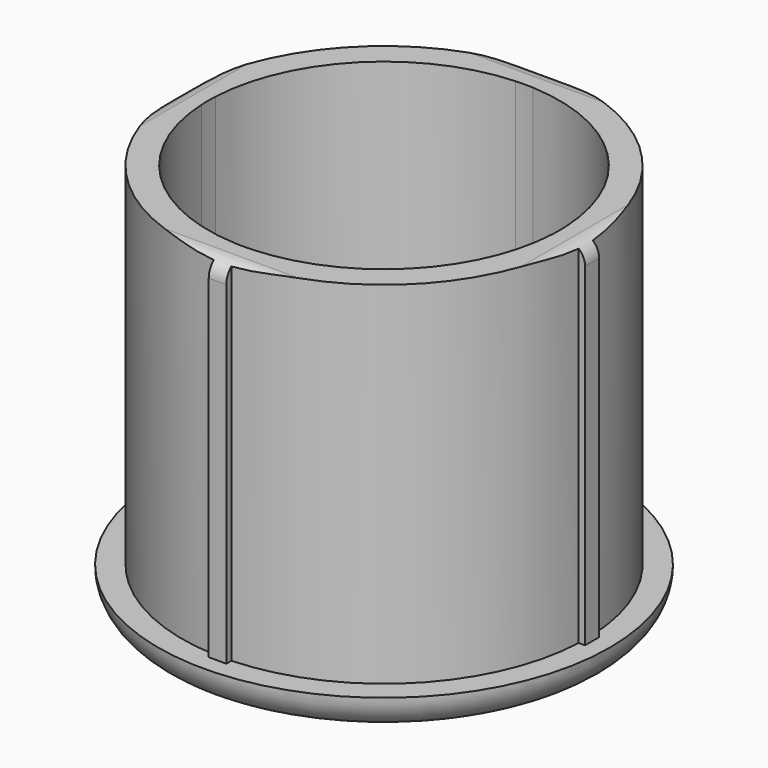
from build123d import *

# Parameters (mm, degrees)
F0_R     = 12.85
F1_DEPTH = 2
F3_DEPTH = 20
F4_R     = 1
F5_R     = 1.99999


# Not quite as in the source:
# - a fillet or chamfer is up to 0.001 mm smaller than in the source, because OpenCascade refuses the exact size


with BuildPart() as f1:
    # F0 (on Top) → F1 (new body)
    with BuildSketch(Plane.XY):
        Circle(F0_R)
    extrude(amount=F1_DEPTH)

    # F2 (on face) → F3 (join)
    with BuildSketch(Plane.XY.offset(2)):
        with BuildLine():
            ThreePointArc((11.4891252931, -0.5), (11.4972810018, -0.2500591226), (11.5, 0))
            ThreePointArc((11.5, 0), (11.4972810018, 0.2500591226), (11.4891252931, 0.5))
            Line((11.4891252931, 0.5), (9.9874921777, 0.5))
            ThreePointArc((9.9874921777, 0.5), (9.9968725554, 0.2500782106), (10, 0))
            ThreePointArc((10, 0), (9.9968725554, -0.2500782106), (9.9874921777, -0.5))
            Line((9.9874921777, -0.5), (11.4891252931, -0.5))
        make_face()
        with BuildLine():
            ThreePointArc((11.4891252931, 0.5), (11.4972810018, 0.2500591226), (11.5, 0))
            ThreePointArc((11.5, 0), (11.4972810018, -0.2500591226), (11.4891252931, -0.5))
            Line((11.4891252931, -0.5), (11.85, -0.5))
            Line((11.85, -0.5), (11.85, 0.5))
            Line((11.85, 0.5), (11.4891252931, 0.5))
        make_face()
        with BuildLine():
            Line((9.9874921777, 0.5), (11.4891252931, 0.5))
            ThreePointArc((11.4891252931, 0.5), (8.1317279836, 8.1317279836), (0.5, 11.4891252931))
            Line((0.5, 11.4891252931), (0.5, 9.9874921777))
            ThreePointArc((0.5, 9.9874921777), (7.0710678119, 7.0710678119), (9.9874921777, 0.5))
        make_face()
        with BuildLine():
            ThreePointArc((0.5, -11.4891252931), (8.1317279836, -8.1317279836), (11.4891252931, -0.5))
            Line((11.4891252931, -0.5), (9.9874921777, -0.5))
            ThreePointArc((9.9874921777, -0.5), (7.0710678119, -7.0710678119), (0.5, -9.9874921777))
            Line((0.5, -9.9874921777), (0.5, -11.4891252931))
        make_face()
        with BuildLine():
            Line((0.5, 9.9874921777), (0.5, 11.4891252931))
            ThreePointArc((0.5, 11.4891252931), (0, 11.5), (-0.5, 11.4891252931))
            Line((-0.5, 11.4891252931), (-0.5, 9.9874921777))
            ThreePointArc((-0.5, 9.9874921777), (0, 10), (0.5, 9.9874921777))
        make_face()
        with BuildLine():
            ThreePointArc((-0.5, 11.4891252931), (0, 11.5), (0.5, 11.4891252931))
            Line((0.5, 11.4891252931), (0.5, 11.85))
            Line((0.5, 11.85), (-0.5, 11.85))
            Line((-0.5, 11.85), (-0.5, 11.4891252931))
        make_face()
        with BuildLine():
            Line((0.5, -11.85), (0.5, -11.4891252931))
            ThreePointArc((0.5, -11.4891252931), (0, -11.5), (-0.5, -11.4891252931))
            Line((-0.5, -11.4891252931), (-0.5, -11.85))
            Line((-0.5, -11.85), (0.5, -11.85))
        make_face()
        with BuildLine():
            ThreePointArc((-0.5, -11.4891252931), (0, -11.5), (0.5, -11.4891252931))
            Line((0.5, -11.4891252931), (0.5, -9.9874921777))
            ThreePointArc((0.5, -9.9874921777), (0, -10), (-0.5, -9.9874921777))
            Line((-0.5, -9.9874921777), (-0.5, -11.4891252931))
        make_face()
        with BuildLine():
            Line((-0.5, 9.9874921777), (-0.5, 11.4891252931))
            ThreePointArc((-0.5, 11.4891252931), (-8.1317279836, 8.1317279836), (-11.4891252931, 0.5))
            Line((-11.4891252931, 0.5), (-9.9874921777, 0.5))
            ThreePointArc((-9.9874921777, 0.5), (-7.0710678119, 7.0710678119), (-0.5, 9.9874921777))
        make_face()
        with BuildLine():
            ThreePointArc((-11.4891252931, -0.5), (-8.1317279836, -8.1317279836), (-0.5, -11.4891252931))
            Line((-0.5, -11.4891252931), (-0.5, -9.9874921777))
            ThreePointArc((-0.5, -9.9874921777), (-7.0710678119, -7.0710678119), (-9.9874921777, -0.5))
            Line((-9.9874921777, -0.5), (-11.4891252931, -0.5))
        make_face()
        with BuildLine():
            Line((-9.9874921777, 0.5), (-11.4891252931, 0.5))
            ThreePointArc((-11.4891252931, 0.5), (-11.5, 0), (-11.4891252931, -0.5))
            Line((-11.4891252931, -0.5), (-9.9874921777, -0.5))
            ThreePointArc((-9.9874921777, -0.5), (-10, 0), (-9.9874921777, 0.5))
        make_face()
        with BuildLine():
            ThreePointArc((-11.4891252931, -0.5), (-11.5, 0), (-11.4891252931, 0.5))
            Line((-11.4891252931, 0.5), (-11.85, 0.5))
            Line((-11.85, 0.5), (-11.85, -0.5))
            Line((-11.85, -0.5), (-11.4891252931, -0.5))
        make_face()
    extrude(amount=F3_DEPTH)

    # F4
    f4_edges = [f1.edges().sort_by_distance(p)[0] for p in [
        (11.85, 0, 22),
        (0, 11.85, 22),
        (-11.85, 0, 22),
        (0, -11.85, 22),
    ]]
    fillet(f4_edges, radius=F4_R)

    # F5 (radius 2 in the source; OpenCascade refuses exactly that, so slightly less here)
    f5_edges = [f1.edges().sort_by_distance(p)[0] for p in [
        (-12.85, 0, 0),
    ]]
    fillet(f5_edges, radius=F5_R)


solid = f1.part
